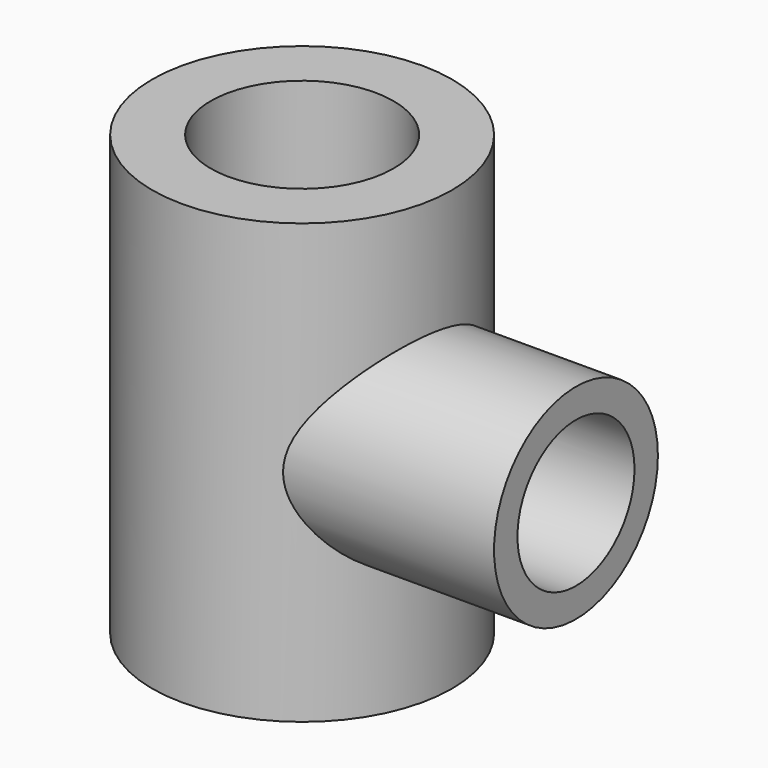
from build123d import *

# Parameters (mm, degrees)
F0_R          = 13.0175
F0_R_2        = 7.9375
F1_DEPTH      = 19.05
F1_DEPTH_BACK = 19.05
F4_END_RADIUS = 13.0175
F3_R          = 8.89
F3_R_2        = 6.35
F4_REACH      = 63.563217139


with BuildPart() as f1:
    # F0 (on Top) → F1 (new body, two sides)
    with BuildSketch(Plane.XY) as f1_sk:
        with Locations((0, 2.0309128979)):
            Circle(F0_R)
        with Locations((0, 2.0309128979)):
            Circle(F0_R_2, mode=Mode.SUBTRACT)
    extrude(amount=F1_DEPTH)
    extrude(f1_sk.sketch, amount=-F1_DEPTH_BACK)

    f4_end = (Plane(origin=(0, 2.0309128979, -9.525), x_dir=(1, 0, 0), z_dir=(0, 0, 1)) * Cylinder(F4_END_RADIUS, 233.0934565066, mode=Mode.PRIVATE)).faces().sort_by_distance((-13.0175, 2.0309128979, -9.525))[0]
    # F3 (on offset) → F4 (join, up to the whole of a round face its end follows)
    with BuildSketch(Plane.YZ.offset(25.4)):
        Circle(F3_R)
        Circle(F3_R_2, mode=Mode.SUBTRACT)
    f4_long = extrude(amount=-F4_REACH, mode=Mode.PRIVATE)
    add(split(f4_long, bisect_by=f4_end, keep=Keep.ALL, mode=Mode.PRIVATE).solids().sort_by_distance((25.4, -8.6385528286, 0))[0])


solid = f1.part
